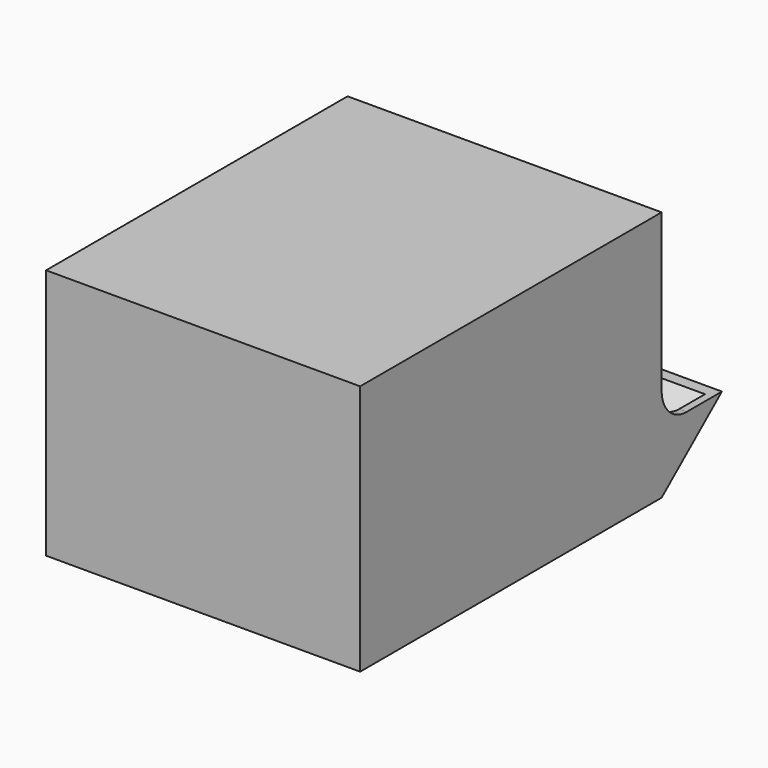
from build123d import *

# Parameters (mm, degrees)
F1_DEPTH = 25
F2_T     = -1.2
F3_R     = 20
F4_R     = 5


with BuildPart() as f1:
    # F0 (on Right) → F1 (new body, symmetric)
    with BuildSketch(Plane.YZ):
        Polygon((30, -10), (30, 20), (-30, 20), (-30, -20), (30, -20), align=None)
        Polygon((42, -10), (30, -10), (30, -20), align=None)
    extrude(amount=F1_DEPTH, both=True)

    # F2
    f2_openings = [f1.faces().sort_by_distance(p)[0] for p in [
        (0, 30, 5),
        (0, 36, -10),
    ]]
    offset(amount=F2_T, openings=f2_openings)

    # F3
    f3_edges = [f1.edges().sort_by_distance(p)[0] for p in [
        (0, 29.56554, -18.8),
    ]]
    fillet(f3_edges, radius=F3_R)

    # F4
    f4_edges = [f1.edges().sort_by_distance(p)[0] for p in [
        (-24.4, 30, -10),
        (24.4, 30, -10),
    ]]
    fillet(f4_edges, radius=F4_R)


solid = f1.part
